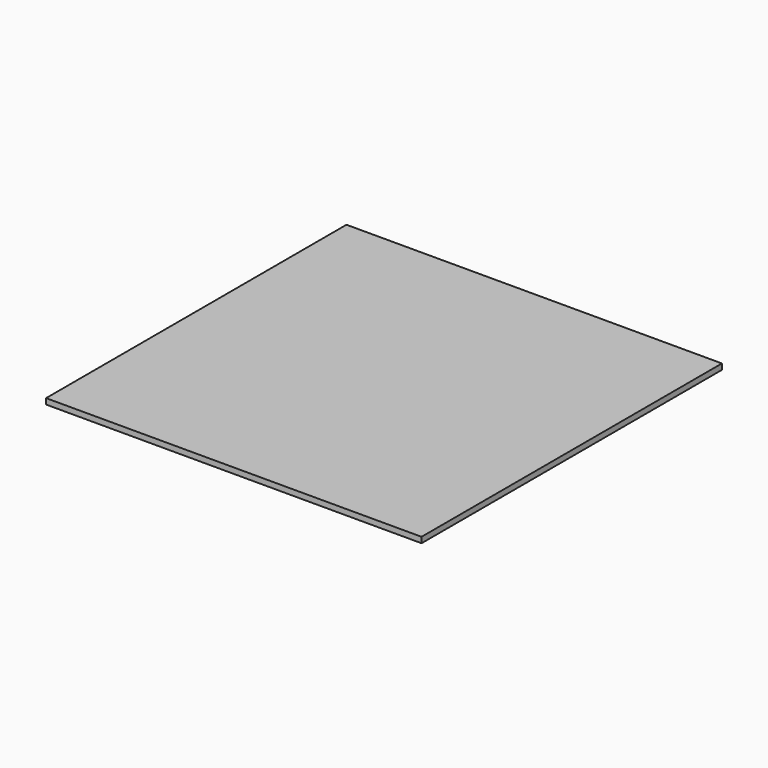
from build123d import *

# Parameters (mm, degrees)
F0_W     = 838.2
F0_H     = 838.2
F1_DEPTH = 12.7


# Not quite as in the source:
# - a length typed as a fraction of an inch, garbled in the dataset ("3 / 203.2 mm" for 3/8 in), is restored


with BuildPart() as f1:
    # F0 (on Top) → F1 (new body)
    with BuildSketch(Plane.XY):
        with Locations((-11.2244263291, 89.4415423164)):
            Rectangle(F0_W, F0_H)
    extrude(amount=F1_DEPTH)


solid = f1.part
